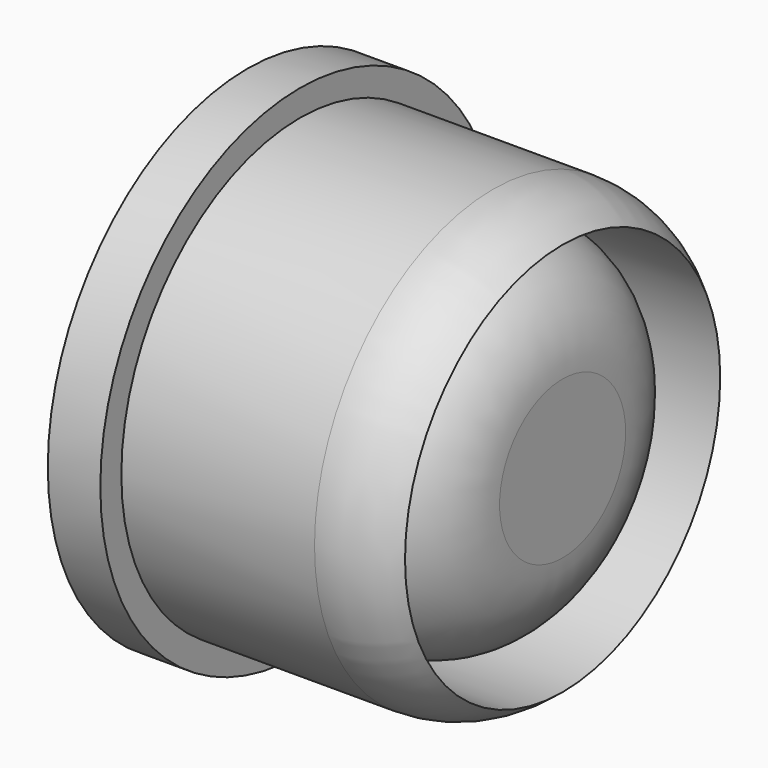
from build123d import *

# Parameters (mm, degrees)
F0_R     = 9.5
F1_DEPTH = 2
F2_R     = 8.5
F3_DEPTH = 10
F4_R     = 7.5
F4_R_2   = 7
F5_DEPTH = 10


# Not quite as in the source:
# - a fillet or chamfer that OpenCascade refuses, or shapes differently, is made with other operations: its cross-section is extruded or revolved along the edge and cut away or added


with BuildPart() as f1:
    # F0 (on Right) → F1 (new body)
    with BuildSketch(Plane.YZ):
        Circle(F0_R)
    extrude(amount=F1_DEPTH)

    # F2 (on face) → F3 (join)
    with BuildSketch(Plane.YZ.offset(2)):
        Circle(F2_R)
    extrude(amount=F3_DEPTH)

    # F4 (on face) → F5 (cut)
    with BuildSketch(Plane.YZ.offset(12)):
        Circle(F4_R)
        Circle(F4_R_2, mode=Mode.SUBTRACT)
    extrude(amount=-F5_DEPTH, mode=Mode.SUBTRACT)

    # F6: fillet of radius 4 on 2 edges, made by hand

    # F6_s1 → F6_t2 (revolve, cut)
    with BuildSketch(Plane.XY):
        with BuildLine():
            ThreePointArc((8, 7), (10.8284271247, 5.8284271247), (12, 3))
            Line((12, 3), (12, 7))
            Line((12, 7), (8, 7))
        make_face()
    revolve(axis=Axis((12, 0, 0), (1, 0, 0)), mode=Mode.SUBTRACT)

    # F6_s3 → F6_t4 (revolve, cut)
    with BuildSketch(Plane.XY):
        with BuildLine():
            ThreePointArc((9.3542486889, 8.5), (10.7684622513, 8.2416573868), (12, 7.5))
            Line((12, 7.5), (12, 8.5))
            Line((12, 8.5), (9.3542486889, 8.5))
        make_face()
    revolve(axis=Axis((12, 0, 0), (1, 0, 0)), mode=Mode.SUBTRACT)


solid = f1.part
